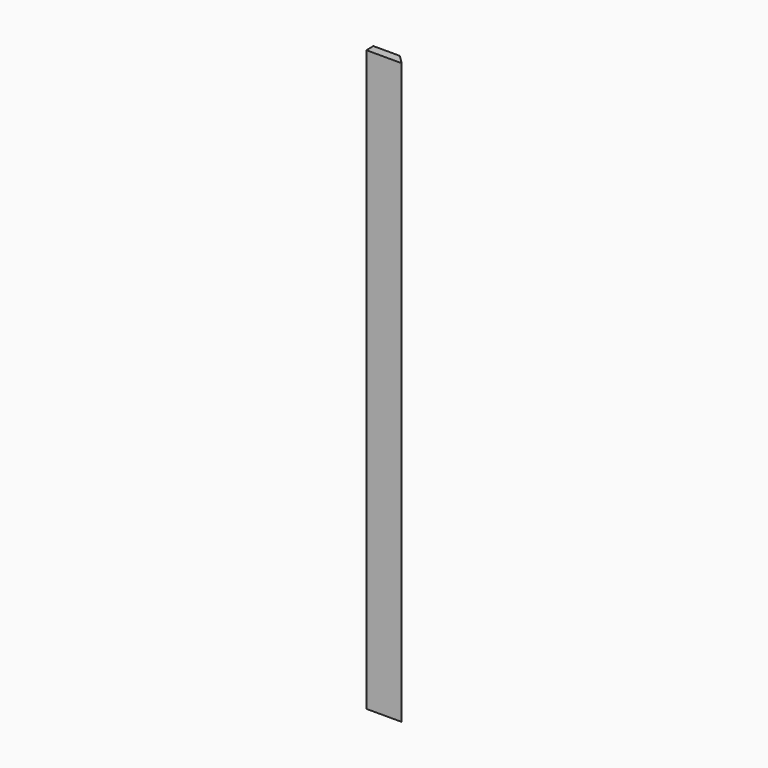
from build123d import *

# Parameters (mm, degrees)
F0_W     = 76.2
F0_H     = 19.05
F1_DEPTH = 625.475
F2_SIZE2 = 19.04999
F2_SIZE  = 19.04999


# Not quite as in the source:
# - a fillet or chamfer is up to 0.001 mm smaller than in the source, because OpenCascade refuses the exact size


with BuildPart() as f1:
    # F0 (on Top) → F1 (new body, symmetric)
    with BuildSketch(Plane.XY):
        Rectangle(F0_W, F0_H)
    extrude(amount=F1_DEPTH, both=True)

    # F2 (size 19.05 and 19.05 in the source; OpenCascade refuses exactly that, so slightly less here)
    f2_edges = [f1.edges().sort_by_distance(p)[0] for p in [
        (38.1, 9.525, 0),
    ]]
    chamfer(f2_edges, length=F2_SIZE, length2=F2_SIZE2)


solid = f1.part
